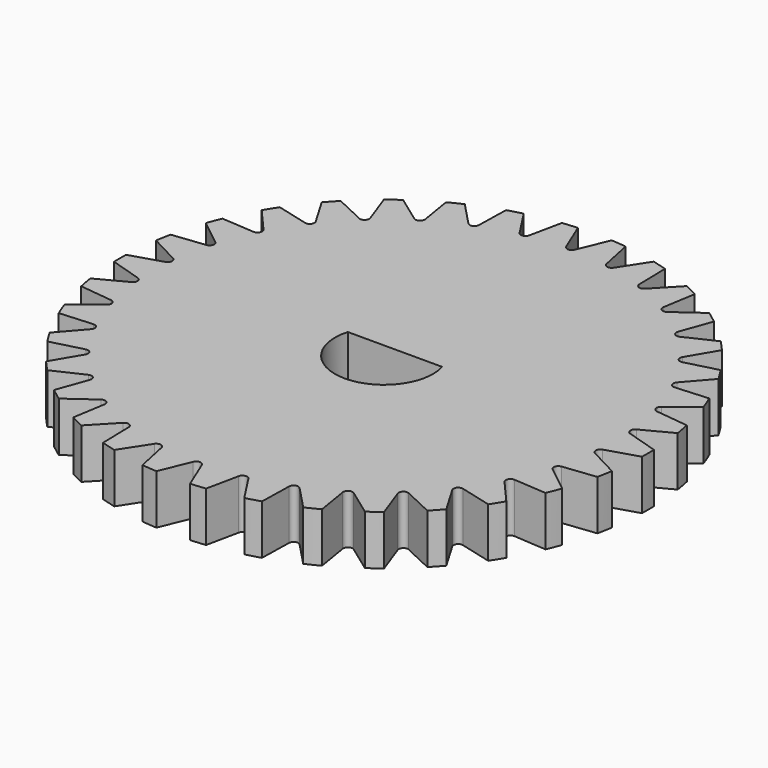
from build123d import *

# Parameters (mm, degrees)
F0_R            = 16.8606013276
F1_DEPTH        = 3.175
F3_DEPTH        = 3.175
F3_COPIES_COUNT = 34


# Not quite as in the source:
# - a pattern or mirror of a feature is missing from the dataset's text; its kind, count and spacing are read off the source's solid
# - a feature names something its author has since deleted; it is built from what else it names


with BuildPart() as f1:
    # F0 (on Top) → F1 (new body)
    with BuildSketch(Plane.XY):
        Circle(F0_R)
        with BuildLine():
            ThreePointArc((3.0120209, 0.8762828927), (0, -3.1369), (-3.0120209, 0.8762828927))
            Line((-3.0120209, 0.8762828927), (3.0120209, 0.8762828927))
        make_face(mode=Mode.SUBTRACT)
    extrude(amount=F1_DEPTH)

    # F2 (on face) → F3 (cut, through all)
    with BuildSketch(Plane.XY.offset(3.175)):
        with BuildLine():
            Line((0.2750051008, 14.882965874), (1.0776094804, 16.8261295293))
            ThreePointArc((1.0776094804, 16.8261295293), (0, 16.8606013276), (-1.0776094804, 16.8261295293))
            Line((-1.0776094804, 16.8261295293), (-0.2750051008, 14.882965874))
            ThreePointArc((-0.2750051008, 14.882965874), (0, 14.6990139664), (0.2750051008, 14.882965874))
        make_face()
    f3 = extrude(amount=-F3_DEPTH, mode=Mode.SUBTRACT)

    # F3_copies: F3 ×34 about axis
    f3_copies_axis = Axis((0, 0, 0), (0, 0, 1))
    for i in range(1, F3_COPIES_COUNT):
        add(f3.rotate(f3_copies_axis, i * 360 / F3_COPIES_COUNT), mode=Mode.SUBTRACT)


solid = f1.part
